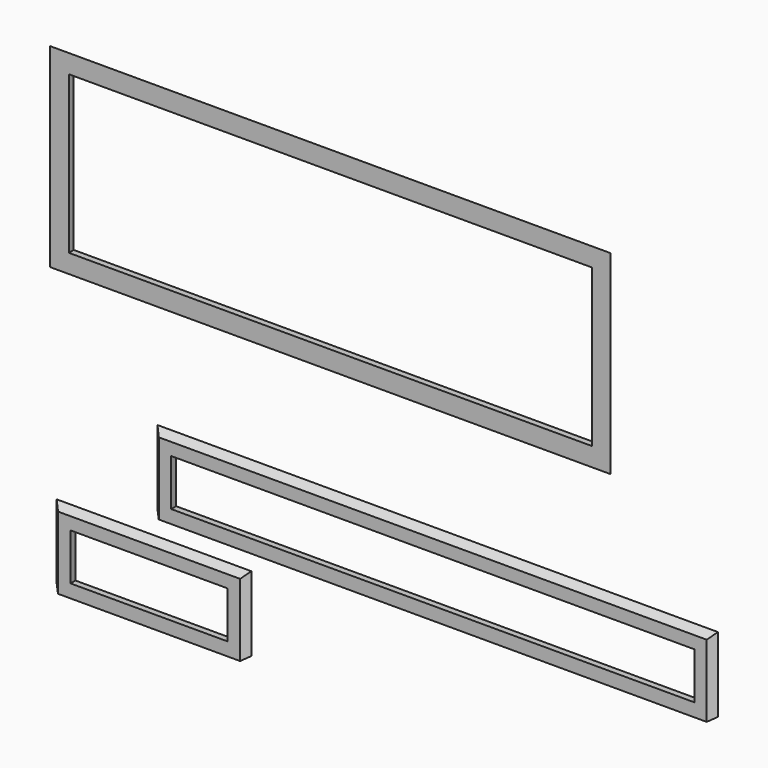
from build123d import *

# Parameters (mm, degrees)
F0_W      = 672
F0_H      = 24
F0_W_2    = 24
F0_H_2    = 60
F0_H_3    = 12
F1_DEPTH  = 8
F3_DEPTH  = 720
F4_SIZE   = 7.99999
F5_W      = 202
F5_H      = 24
F5_W_2    = 24
F5_H_2    = 60
F5_H_3    = 12
F6_DEPTH  = 8
F8_DEPTH  = 250
F9_SIZE   = 7.99999
F10_W     = 720
F10_H     = 250
F11_DEPTH = 8
F12_SIZE  = 7.99999
F13_W     = 672
F13_H     = 202
F14_DEPTH = 25


# Not quite as in the source:
# - a fillet or chamfer is up to 0.001 mm smaller than in the source, because OpenCascade refuses the exact size


with BuildPart() as f1:
    # F0 (on Front) → F1 (new body)
    with BuildSketch(Plane.XZ):
        with Locations((194.5052774136, 36.6904993206)):
            Rectangle(F0_W, F0_H)
        with Locations((-153.4947225864, 36.6904993206)):
            Rectangle(F0_W_2, F0_H)
        with Locations((-153.4947225864, -5.3095006794)):
            Rectangle(F0_W_2, F0_H_2)
        with Locations((-153.4947225864, -41.3095006794)):
            Rectangle(F0_W_2, F0_H_3)
        with Locations((194.5052774136, -41.3095006794)):
            Rectangle(F0_W, F0_H_3)
        with Locations((542.5052774136, -5.3095006794)):
            Rectangle(F0_W_2, F0_H_2)
        with Locations((542.5052774136, 36.6904993206)):
            Rectangle(F0_W_2, F0_H)
        with Locations((542.5052774136, -41.3095006794)):
            Rectangle(F0_W_2, F0_H_3)
    extrude(amount=F1_DEPTH)

    # F2 (on face) → F3 (join)
    with BuildSketch(Plane(origin=(-165.4947225864, 0, 0), x_dir=(0, -1, 0), z_dir=(-1, 0, 0))):
        Polygon((8, -52.3095006794), (8, -47.3095006794), (0, -47.3095006794), align=None)
    extrude(amount=-F3_DEPTH)

    # F4 (size 8 in the source; OpenCascade refuses exactly that, so slightly less here)
    f4_edges = [f1.edges().sort_by_distance(p)[0] for p in [
        (554.505277, -8, -1.809501),
        (194.505277, -8, 48.690499),
        (-165.494723, -8, -1.809501),
    ]]
    chamfer(f4_edges, length=F4_SIZE)


with BuildPart() as f6:
    # F5 (on Front) → F6 (new body)
    with BuildSketch(Plane.XZ):
        with Locations((-169.9683964583, -89.4514269531)):
            Rectangle(F5_W, F5_H)
        with Locations((-282.9683964583, -89.4514269531)):
            Rectangle(F5_W_2, F5_H)
        with Locations((-282.9683964583, -131.4514269531)):
            Rectangle(F5_W_2, F5_H_2)
        with Locations((-282.9683964583, -167.4514269531)):
            Rectangle(F5_W_2, F5_H_3)
        with Locations((-169.9683964583, -167.4514269531)):
            Rectangle(F5_W, F5_H_3)
        with Locations((-56.9683964583, -167.4514269531)):
            Rectangle(F5_W_2, F5_H_3)
        with Locations((-56.9683964583, -131.4514269531)):
            Rectangle(F5_W_2, F5_H_2)
        with Locations((-56.9683964583, -89.4514269531)):
            Rectangle(F5_W_2, F5_H)
    extrude(amount=F6_DEPTH)

    # F7 (on face) → F8 (join)
    with BuildSketch(Plane(origin=(-294.9683964583, 0, 0), x_dir=(0, -1, 0), z_dir=(-1, 0, 0))):
        Polygon((8, -178.4514269531), (8, -173.4514269531), (0, -173.4514269531), align=None)
    extrude(amount=-F8_DEPTH)

    # F9 (size 8 in the source; OpenCascade refuses exactly that, so slightly less here)
    f9_edges = [f6.edges().sort_by_distance(p)[0] for p in [
        (-169.968396, -8, -77.451427),
        (-294.968396, -8, -127.951427),
        (-44.968396, -8, -127.951427),
    ]]
    chamfer(f9_edges, length=F9_SIZE)


with BuildPart() as f11:
    # F10 (on Front) → F11 (new body)
    with BuildSketch(Plane.XZ):
        with Locations((56.4652234316, 307.4194252866)):
            Rectangle(F10_W, F10_H)
    extrude(amount=-F11_DEPTH)

    # F12 (size 8 in the source; OpenCascade refuses exactly that, so slightly less here)
    f12_edges = [f11.edges().sort_by_distance(p)[0] for p in [
        (56.465223, 8, 182.419425),
        (416.465223, 8, 307.419425),
        (56.465223, 8, 432.419425),
        (-303.534777, 8, 307.419425),
    ]]
    chamfer(f12_edges, length=F12_SIZE)

    # F13 (on face) → F14 (cut)
    with BuildSketch(Plane.XZ):
        with Locations((56.4652234316, 307.4194252866)):
            Rectangle(F13_W, F13_H)
    extrude(amount=-F14_DEPTH, mode=Mode.SUBTRACT)


solid = Compound([f1.part, f6.part, f11.part])
